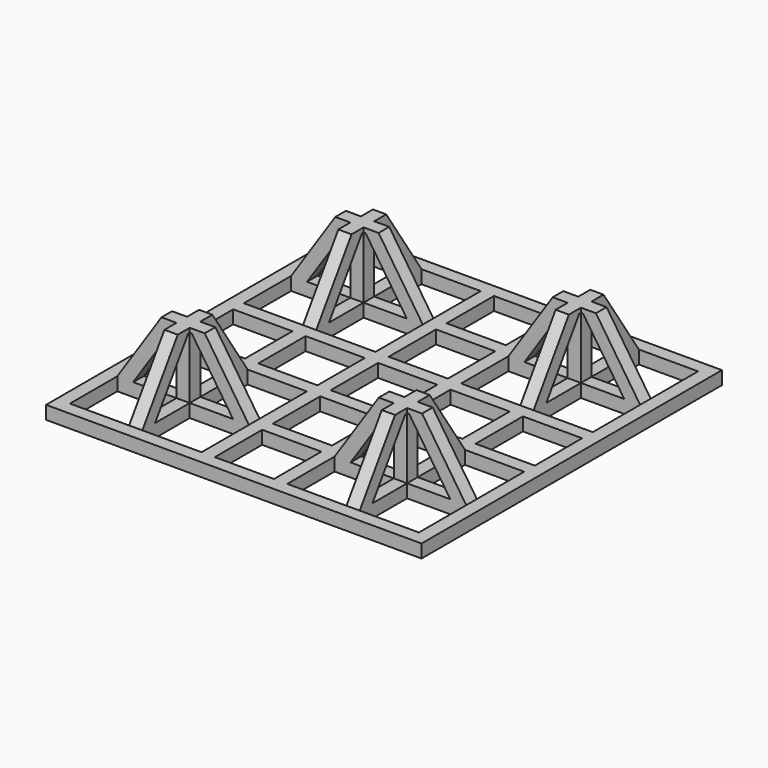
from build123d import *

# Parameters (mm, degrees)
F0_W       = 85
F0_H       = 85
F1_DEPTH   = 3
F2_W       = 13.4
F2_H       = 13.4
F3_DEPTH   = 25
F5_DEPTH   = 15
F6_SIZE2   = 14.99999
F6_SIZE    = 9.99999
F6_2_SIZE2 = 14.99999
F6_2_SIZE  = 9.99999
F6_3_SIZE2 = 14.99999
F6_3_SIZE  = 9.99999
F6_4_SIZE2 = 14.99999
F6_4_SIZE  = 9.99999
F7_SIZE2   = 9.99999
F7_SIZE    = 14.99999
F7_2_SIZE2 = 9.99999
F7_2_SIZE  = 14.99999
F7_3_SIZE2 = 9.99999
F7_3_SIZE  = 14.99999
F7_4_SIZE2 = 9.99999
F7_4_SIZE  = 14.99999
F7_5_SIZE2 = 9.99999
F7_5_SIZE  = 14.99999
F9_DEPTH   = 68.601
F11_DEPTH  = 68.601


# Not quite as in the source:
# - a fillet or chamfer is up to 0.001 mm smaller than in the source, because OpenCascade refuses the exact size
# - a feature names something its author has since deleted; it is built from what else it names


with BuildPart() as f1:
    # F0 (on Top) → F1 (new body)
    with BuildSketch(Plane.XY):
        Rectangle(F0_W, F0_H)
    extrude(amount=F1_DEPTH)

    # F2 (on face) → F3 (cut)
    with BuildSketch(Plane.XY.offset(3)):
        with Locations((-32.8, 16.4)):
            Rectangle(F2_W, F2_H)
        with Locations((-32.8, 0)):
            Rectangle(F2_W, F2_H)
        with Locations((-32.8, -16.4)):
            Rectangle(F2_W, F2_H)
        with Locations((-32.8, -32.8)):
            Rectangle(F2_W, F2_H)
        with Locations((-16.4, 32.8)):
            Rectangle(F2_W, F2_H)
        with Locations((-16.4, 16.4)):
            Rectangle(F2_W, F2_H)
        with Locations((-16.4, 0)):
            Rectangle(F2_W, F2_H)
        with Locations((-16.4, -16.4)):
            Rectangle(F2_W, F2_H)
        with Locations((-16.4, -32.8)):
            Rectangle(F2_W, F2_H)
        with Locations((0, 32.8)):
            Rectangle(F2_W, F2_H)
        with Locations((0, 16.4)):
            Rectangle(F2_W, F2_H)
        Rectangle(F2_W, F2_H)
        with Locations((0, -16.4)):
            Rectangle(F2_W, F2_H)
        with Locations((0, -32.8)):
            Rectangle(F2_W, F2_H)
        with Locations((16.4, 32.8)):
            Rectangle(F2_W, F2_H)
        with Locations((16.4, 16.4)):
            Rectangle(F2_W, F2_H)
        with Locations((16.4, 0)):
            Rectangle(F2_W, F2_H)
        with Locations((16.4, -16.4)):
            Rectangle(F2_W, F2_H)
        with Locations((16.4, -32.8)):
            Rectangle(F2_W, F2_H)
        with Locations((32.8, 32.8)):
            Rectangle(F2_W, F2_H)
        with Locations((32.8, 16.4)):
            Rectangle(F2_W, F2_H)
        with Locations((32.8, 0)):
            Rectangle(F2_W, F2_H)
        with Locations((32.8, -16.4)):
            Rectangle(F2_W, F2_H)
        with Locations((32.8, -32.8)):
            Rectangle(F2_W, F2_H)
        with Locations((-32.8, 32.8)):
            Rectangle(F2_W, F2_H)
    extrude(amount=-F3_DEPTH, mode=Mode.SUBTRACT)

    # F4 (on face) → F5 (join)
    with BuildSketch(Plane.XY.offset(3)):
        Polygon((-23.1, -9.7), (-26.1, -9.7), (-26.1, -23.1), (-39.5, -23.1), (-39.5, -26.1), (-26.1, -26.1), (-26.1, -39.5), (-23.1, -39.5), (-23.1, -26.1), (-9.7, -26.1), (-9.7, -23.1), (-23.1, -23.1), align=None)
        Polygon((-9.7, 23.1), (-9.7, 26.1), (-23.1, 26.1), (-23.1, 39.5), (-26.1, 39.5), (-26.1, 26.1), (-39.5, 26.1), (-39.5, 23.1), (-26.1, 23.1), (-26.1, 9.7), (-23.1, 9.7), (-23.1, 23.1), align=None)
        Polygon((26.1, 26.1), (26.1, 39.5), (23.1, 39.5), (23.1, 26.1), (9.7, 26.1), (9.7, 23.1), (23.1, 23.1), (23.1, 9.7), (26.1, 9.7), (26.1, 23.1), (39.5, 23.1), (39.5, 26.1), align=None)
        Polygon((26.1, -23.1), (26.1, -9.7), (23.1, -9.7), (23.1, -23.1), (9.7, -23.1), (9.7, -26.1), (23.1, -26.1), (23.1, -39.5), (26.1, -39.5), (26.1, -26.1), (39.5, -26.1), (39.5, -23.1), align=None)
    extrude(amount=F5_DEPTH)

    # F6 (size 10 and 15 in the source; OpenCascade refuses exactly that, so slightly less here)
    f6_edges = [f1.edges().sort_by_distance(p)[0] for p in [
        (-39.5, -24.6, 18),
        (-24.6, -9.7, 18),
        (-9.7, -24.6, 18),
        (-24.6, -39.5, 18),
    ]]
    f6_side = f1.faces().sort_by_distance((-24.6, -24.6, 18))[0]
    chamfer(f6_edges, length=F6_SIZE, length2=F6_SIZE2, reference=f6_side)

    # F6#2 (size 10 and 15 in the source; OpenCascade refuses exactly that, so slightly less here)
    f6_2_edges = [f1.edges().sort_by_distance(p)[0] for p in [
        (-39.5, 24.6, 18),
        (-24.6, 39.5, 18),
    ]]
    f6_2_side = f1.faces().sort_by_distance((-24.6, 24.6, 18))[0]
    chamfer(f6_2_edges, length=F6_2_SIZE, length2=F6_2_SIZE2, reference=f6_2_side)

    # F6#3 (size 10 and 15 in the source; OpenCascade refuses exactly that, so slightly less here)
    f6_3_edges = [f1.edges().sort_by_distance(p)[0] for p in [
        (9.7, 24.6, 18),
        (24.6, 39.5, 18),
    ]]
    f6_3_side = f1.faces().sort_by_distance((24.6, 24.6, 18))[0]
    chamfer(f6_3_edges, length=F6_3_SIZE, length2=F6_3_SIZE2, reference=f6_3_side)

    # F6#4 (size 10 and 15 in the source; OpenCascade refuses exactly that, so slightly less here)
    f6_4_edges = [f1.edges().sort_by_distance(p)[0] for p in [
        (24.6, -9.7, 18),
        (9.7, -24.6, 18),
        (39.5, -24.6, 18),
    ]]
    f6_4_side = f1.faces().sort_by_distance((24.6, -24.6, 18))[0]
    chamfer(f6_4_edges, length=F6_4_SIZE, length2=F6_4_SIZE2, reference=f6_4_side)

    # F7 (size 15 and 10 in the source; OpenCascade refuses exactly that, so slightly less here)
    f7_edges = [f1.edges().sort_by_distance(p)[0] for p in [
        (-9.7, 24.6, 18),
    ]]
    f7_side = f1.faces().sort_by_distance((-9.7, 24.6, 10.5))[0]
    chamfer(f7_edges, length=F7_SIZE, length2=F7_SIZE2, reference=f7_side)

    # F7#2 (size 15 and 10 in the source; OpenCascade refuses exactly that, so slightly less here)
    f7_2_edges = [f1.edges().sort_by_distance(p)[0] for p in [
        (-24.6, 9.7, 18),
    ]]
    f7_2_side = f1.faces().sort_by_distance((-24.6, 9.7, 10.5))[0]
    chamfer(f7_2_edges, length=F7_2_SIZE, length2=F7_2_SIZE2, reference=f7_2_side)

    # F7#3 (size 15 and 10 in the source; OpenCascade refuses exactly that, so slightly less here)
    f7_3_edges = [f1.edges().sort_by_distance(p)[0] for p in [
        (24.6, 9.7, 18),
    ]]
    f7_3_side = f1.faces().sort_by_distance((24.6, 9.7, 10.5))[0]
    chamfer(f7_3_edges, length=F7_3_SIZE, length2=F7_3_SIZE2, reference=f7_3_side)

    # F7#4 (size 15 and 10 in the source; OpenCascade refuses exactly that, so slightly less here)
    f7_4_edges = [f1.edges().sort_by_distance(p)[0] for p in [
        (39.5, 24.6, 18),
    ]]
    f7_4_side = f1.faces().sort_by_distance((39.5, 24.6, 10.5))[0]
    chamfer(f7_4_edges, length=F7_4_SIZE, length2=F7_4_SIZE2, reference=f7_4_side)

    # F7#5 (size 15 and 10 in the source; OpenCascade refuses exactly that, so slightly less here)
    f7_5_edges = [f1.edges().sort_by_distance(p)[0] for p in [
        (24.6, -39.5, 18),
    ]]
    f7_5_side = f1.faces().sort_by_distance((24.6, -39.5, 10.5))[0]
    chamfer(f7_5_edges, length=F7_5_SIZE, length2=F7_5_SIZE2, reference=f7_5_side)

    # F8 (on face) → F9 (cut, through all)
    with BuildSketch(Plane.YZ.offset(26.1)):
        Polygon((-26.1, 17), (-26.5611153912, 17), (-35.8944487245, 3), (-26.1, 3), align=None)
        Polygon((-22.6388846088, 17), (-23.1, 17), (-23.1, 3), (-13.3055512755, 3), align=None)
        Polygon((23.1, 17), (22.6388846088, 17), (13.3055512755, 3), (23.1, 3), align=None)
        Polygon((26.5611153912, 17), (26.1, 17), (26.1, 3), (35.8944487245, 3), align=None)
    extrude(amount=-F9_DEPTH, mode=Mode.SUBTRACT)

    # F10 (on face) → F11 (cut, through all)
    with BuildSketch(Plane.XZ.offset(26.1)):
        Polygon((-26.1, 17), (-26.5611153912, 17), (-35.8944487245, 3), (-26.1, 3), align=None)
        Polygon((-22.6388846088, 17), (-23.1, 17), (-23.1, 3), (-13.3055512755, 3), align=None)
        Polygon((23.1, 17), (22.6388846088, 17), (13.3055512755, 3), (23.1, 3), align=None)
        Polygon((26.5611153912, 17), (26.1, 17), (26.1, 3), (35.8944487245, 3), align=None)
    extrude(amount=-F11_DEPTH, mode=Mode.SUBTRACT)


solid = f1.part
